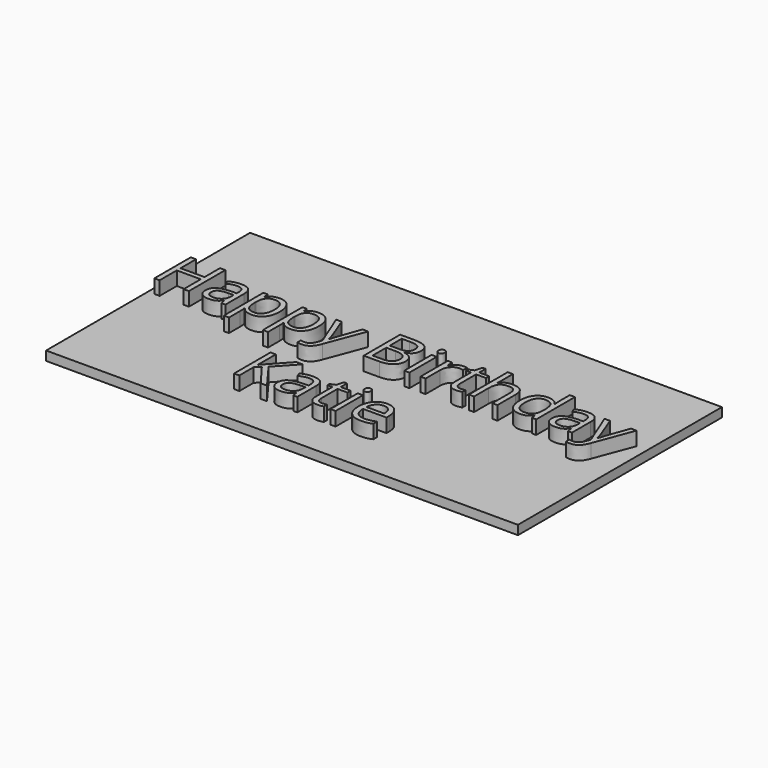
from build123d import *

# Parameters (mm, degrees)
F0_W         = 102.9397919774
F0_H         = 55.6258484721
F1_DEPTH     = 2
F2_TEXT_SIZE = 13.9123824839
F3_DEPTH     = 3


# Not quite as in the source:
# - Text() gives the source's letters only with a copy of the font that has no kerning and outlines rounded to 1/6400 em; it was checked with that copy


with BuildPart() as f1:
    # F0 (on Top) → F1 (new body)
    with BuildSketch(Plane.XY):
        with Locations((1.1721923947, -2.7706362307)):
            Rectangle(F0_W, F0_H)
    extrude(amount=F1_DEPTH)

    # F2 (on face) → F3 (join)
    with BuildSketch(Plane.XY.offset(2)):
        with Locations((-50.297703594, -2.7706362307)):
            Text('Happy Birthday', F2_TEXT_SIZE, font='Open Sans', text_align=(TextAlign.LEFT, TextAlign.BOTTOM))
        with Locations((-17.7622928695, -21.6914764088)):
            Text('Katie', F2_TEXT_SIZE, font='Open Sans', text_align=(TextAlign.LEFT, TextAlign.BOTTOM))
    extrude(amount=F3_DEPTH)


solid = f1.part
